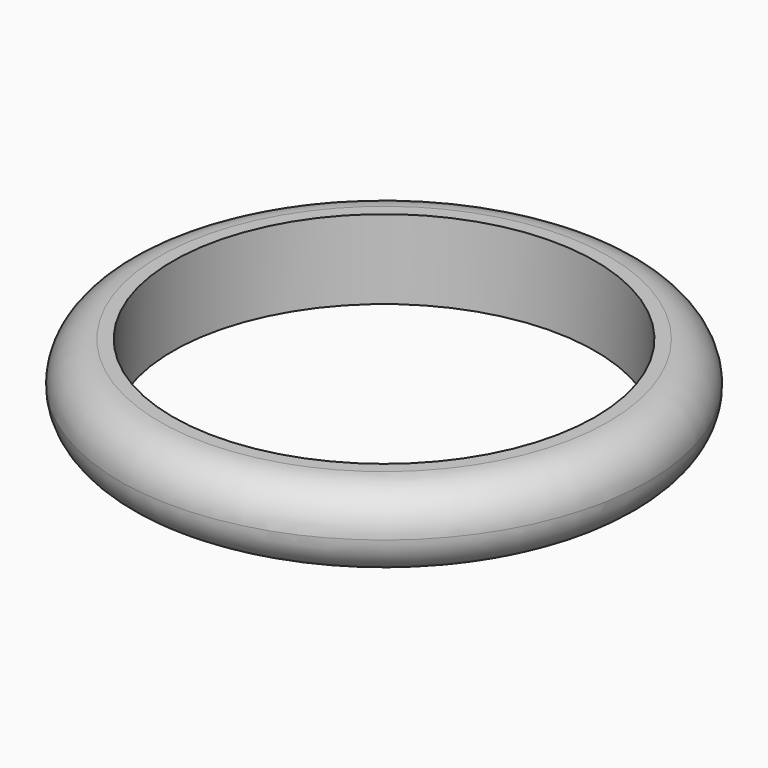
from build123d import *

# Parameters (mm, degrees)
F1_R     = 25.4
F1_R_2   = 20.32
F2_DEPTH = 7.62
F3_R     = 3.81
F0_R     = 3.80999


# Not quite as in the source:
# - a fillet or chamfer is up to 0.001 mm smaller than in the source, because OpenCascade refuses the exact size


with BuildPart() as f2:
    # F1 (on Top) → F2 (new body)
    with BuildSketch(Plane.XY):
        Circle(F1_R)
        Circle(F1_R_2, mode=Mode.SUBTRACT)
    extrude(amount=F2_DEPTH)

    # F3
    f3_edges = [f2.edges().sort_by_distance(p)[0] for p in [
        (-25.4, 0, 0),
    ]]
    fillet(f3_edges, radius=F3_R)

    # F0 (radius 3.81 in the source; OpenCascade refuses exactly that, so slightly less here)
    f0_edges = [f2.edges().sort_by_distance(p)[0] for p in [
        (-25.4, 0, 7.62),
    ]]
    fillet(f0_edges, radius=F0_R)


solid = f2.part
